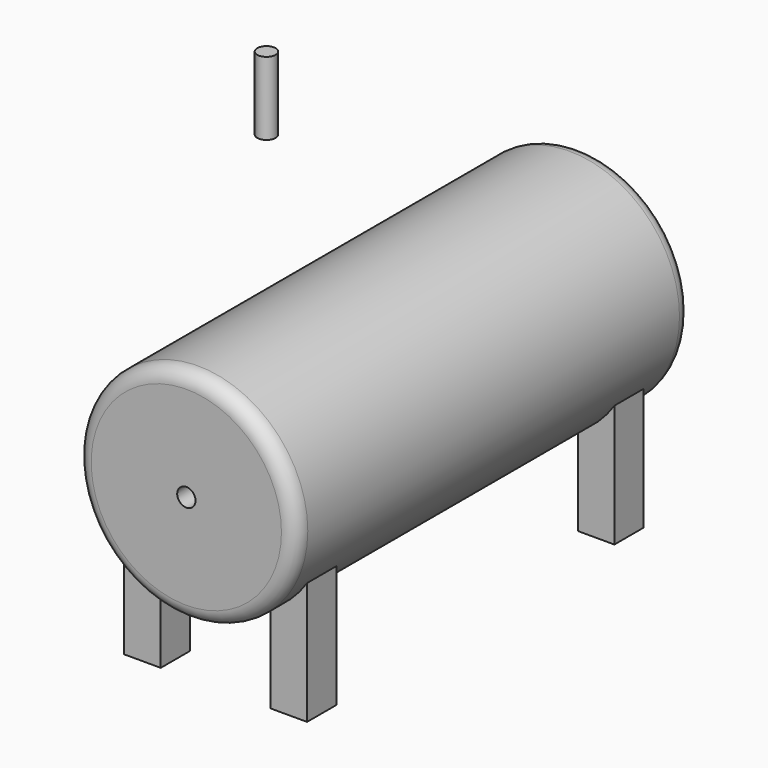
from build123d import *

# Parameters (mm, degrees)
F0_R      = 38.1
F1_DEPTH  = 6.35
F2_R      = 38.1
F2_R_2    = 31.75
F3_DEPTH  = 152.4
F4_R      = 38.1
F4_R_2    = 3.175
F5_DEPTH  = 12.7
F6_R      = 6.35
F7_DEPTH  = 25.4
F8_R      = 5.08
F10_W     = 12.7
F10_H     = 12.7
F10_W_2   = 12.6999954973
F10_R     = 6.35
F11_DEPTH = 25.4
F12_DEPTH = 25.4
F13_DEPTH = 25.4
F15_DEPTH = 25.4
F16_R     = 6.35
F17_DEPTH = 25.4
F18_R     = 3.175
F19_DEPTH = 25.4


with BuildPart() as f1:
    # F0 (on Front) → F1 (new body)
    with BuildSketch(Plane.XZ):
        Circle(F0_R)
    extrude(amount=F1_DEPTH)

    # F2 (on face) → F3 (join)
    with BuildSketch(Plane.XZ.offset(6.35)):
        Circle(F2_R)
        Circle(F2_R_2, mode=Mode.SUBTRACT)
    extrude(amount=F3_DEPTH)

    # F4 (on face) → F5 (join)
    with BuildSketch(Plane.XZ.offset(158.75)):
        Circle(F4_R)
        Circle(F4_R_2, mode=Mode.SUBTRACT)
    extrude(amount=F5_DEPTH)

    # F6 (on face) → F7 (cut)
    with BuildSketch(Plane(origin=(0, 0, 0), x_dir=(-1, 0, 0), z_dir=(0, 1, 0))):
        Circle(F6_R)
    extrude(amount=-F7_DEPTH, mode=Mode.SUBTRACT)

    # F8
    f8_edges = [f1.edges().sort_by_distance(p)[0] for p in [
        (-38.1, 0, 0),
        (-38.1, -171.45, 0),
    ]]
    fillet(f8_edges, radius=F8_R)

    # F10 (on offset) → F11 (join)
    with BuildSketch(Plane.XY.offset(-12.7)):
        with Locations((-25.4, -152.4)):
            Rectangle(F10_W, F10_H)
        with Locations((25.4, -152.4)):
            Rectangle(F10_W, F10_H)
        with Locations((-25.4000022513, -19.05)):
            Rectangle(F10_W_2, F10_H)
        with Locations((25.3999954973, -19.05)):
            Rectangle(F10_W, F10_H)
        with Locations((0, -82.55)):
            Circle(F10_R)
    extrude(amount=-F11_DEPTH)

    # F12 (add): faces of the model
    f12_faces = [f1.faces().sort_by_distance(p)[0] for p in [
        (-25.4, -152.4, -38.1),
        (-25.4000022513, -19.05, -38.1),
        (25.3999954973, -19.05, -38.1),
        (25.4, -152.4, -38.1),
    ]]
    extrude(f12_faces, amount=F12_DEPTH)

    # F13 (add): a face of the model
    f13_faces = [f1.faces().sort_by_distance(p)[0] for p in [
        (0, -82.55, -38.1),
    ]]
    extrude(f13_faces, amount=-F13_DEPTH)

    # F14 (on face) → F15 (join)
    with BuildSketch(Plane(origin=(0, 0, -38.1), x_dir=(1, 0, 0), z_dir=(0, 0, -1))):
        with BuildLine():
            ThreePointArc((-6.743e-07, 88.9), (-6.35, 82.5499993257), (6.743e-07, 76.2))
            ThreePointArc((6.743e-07, 76.2), (6.35, 82.5500006743), (-6.743e-07, 88.9))
        make_face()
    extrude(amount=-F15_DEPTH)

    # F16 (on face) → F17 (cut)
    with BuildSketch(Plane(origin=(0, 0, -38.1), x_dir=(1, 0, 0), z_dir=(0, 0, -1))):
        with Locations((0, 82.55)):
            Circle(F16_R)
    extrude(amount=-F17_DEPTH, mode=Mode.SUBTRACT)


with BuildPart() as f19:
    # F18 (on Top) → F19 (new body)
    with BuildSketch(Plane.XY):
        with Locations((-116.0415932536, 8.3441408351)):
            Circle(F18_R)
    extrude(amount=F19_DEPTH)


solid = Compound([f1.part, f19.part])
